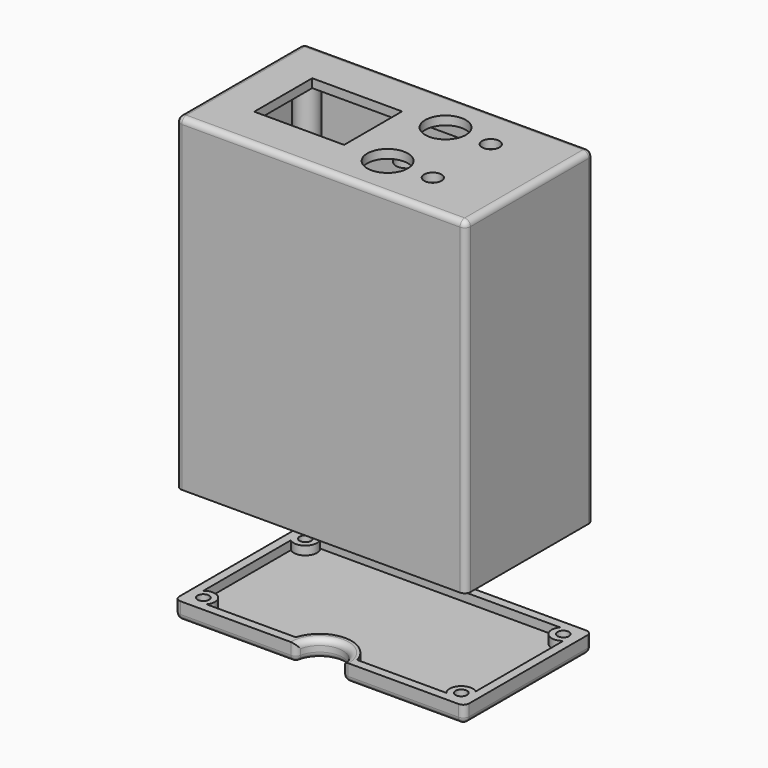
from build123d import *

# Parameters (mm, degrees)
F0_W      = 100
F0_H      = 55
F0_R      = 2.5
F0_R_2    = 7
F0_R_3    = 3
F0_W_2    = 31
F0_H_2    = 25
F1_DEPTH  = 3
F2_DEPTH  = 110
F3_R      = 3.5
F3_R_2    = 1.5
F3_W      = 49.6577308513
F3_H      = 4
F3_R_3    = 1
F4_DEPTH  = 4
F5_R      = 2
F7_R      = 3
F8_DEPTH  = 3
F7_R_2    = 2
F9_DEPTH  = 6
F11_DEPTH = 2.9
F12_R     = 2


# Not quite as in the source:
# - a feature of the source that left no trace in its solid (it failed there, or was rolled back) is left out
# - a feature names something its author has since deleted; it is built from what else it names


with BuildPart() as f1:
    # F0 (on Top) → F1 (new body)
    with BuildSketch(Plane.XY):
        Rectangle(F0_W, F0_H)
        with Locations((-44.5, -22)):
            Circle(F0_R, mode=Mode.SUBTRACT)
        with Locations((44.5, -22)):
            Circle(F0_R, mode=Mode.SUBTRACT)
        with Locations((-44.5, 22)):
            Circle(F0_R, mode=Mode.SUBTRACT)
        with BuildLine():
            ThreePointArc((-47, 18.8775010008), (-41.6715728753, 19.1715728753), (-41.3775010008, 24.5))
            Line((-41.3775010008, 24.5), (41.3775010008, 24.5))
            ThreePointArc((41.3775010008, 24.5), (41.6715728753, 19.1715728753), (47, 18.8775010008))
            Line((47, 18.8775010008), (47, -18.8775010008))
            ThreePointArc((47, -18.8775010008), (41.6715728753, -19.1715728753), (41.3775010008, -24.5))
            Line((41.3775010008, -24.5), (-41.3775010008, -24.5))
            ThreePointArc((-41.3775010008, -24.5), (-41.6715728753, -19.1715728753), (-47, -18.8775010008))
            Line((-47, -18.8775010008), (-47, 18.8775010008))
        make_face(mode=Mode.SUBTRACT)
        with Locations((44.5, 22)):
            Circle(F0_R, mode=Mode.SUBTRACT)
        with BuildLine():
            Line((41.3775010008, 24.5), (-41.3775010008, 24.5))
            ThreePointArc((-41.3775010008, 24.5), (-41.6715728753, 19.1715728753), (-47, 18.8775010008))
            Line((-47, 18.8775010008), (-47, -18.8775010008))
            ThreePointArc((-47, -18.8775010008), (-41.6715728753, -19.1715728753), (-41.3775010008, -24.5))
            Line((-41.3775010008, -24.5), (41.3775010008, -24.5))
            ThreePointArc((41.3775010008, -24.5), (41.6715728753, -19.1715728753), (47, -18.8775010008))
            Line((47, -18.8775010008), (47, 18.8775010008))
            ThreePointArc((47, 18.8775010008), (41.6715728753, 19.1715728753), (41.3775010008, 24.5))
        make_face()
        with Locations((11, -12.5)):
            Circle(F0_R_2, mode=Mode.SUBTRACT)
        with Locations((26.6150971745, -12.5)):
            Circle(F0_R_3, mode=Mode.SUBTRACT)
        with Locations((-19.5, 0)):
            Rectangle(F0_W_2, F0_H_2, mode=Mode.SUBTRACT)
        with Locations((11, 12.5)):
            Circle(F0_R_2, mode=Mode.SUBTRACT)
        with Locations((26.6150971745, 12.5)):
            Circle(F0_R_3, mode=Mode.SUBTRACT)
        with Locations((-44.5, 22)):
            Circle(F0_R)
        with Locations((-44.5, -22)):
            Circle(F0_R)
        with Locations((44.5, -22)):
            Circle(F0_R)
        with Locations((44.5, 22)):
            Circle(F0_R)
    extrude(amount=F1_DEPTH)

    # F0 (on Top) → F2 (join)
    with BuildSketch(Plane.XY):
        Rectangle(F0_W, F0_H)
        with Locations((-44.5, -22)):
            Circle(F0_R, mode=Mode.SUBTRACT)
        with Locations((44.5, -22)):
            Circle(F0_R, mode=Mode.SUBTRACT)
        with Locations((-44.5, 22)):
            Circle(F0_R, mode=Mode.SUBTRACT)
        with BuildLine():
            ThreePointArc((-47, 18.8775010008), (-41.6715728753, 19.1715728753), (-41.3775010008, 24.5))
            Line((-41.3775010008, 24.5), (41.3775010008, 24.5))
            ThreePointArc((41.3775010008, 24.5), (41.6715728753, 19.1715728753), (47, 18.8775010008))
            Line((47, 18.8775010008), (47, -18.8775010008))
            ThreePointArc((47, -18.8775010008), (41.6715728753, -19.1715728753), (41.3775010008, -24.5))
            Line((41.3775010008, -24.5), (-41.3775010008, -24.5))
            ThreePointArc((-41.3775010008, -24.5), (-41.6715728753, -19.1715728753), (-47, -18.8775010008))
            Line((-47, -18.8775010008), (-47, 18.8775010008))
        make_face(mode=Mode.SUBTRACT)
        with Locations((44.5, 22)):
            Circle(F0_R, mode=Mode.SUBTRACT)
    extrude(amount=-F2_DEPTH)

    # F3 (on face) → F4 (join)
    with BuildSketch(Plane.XY):
        with Locations((37, 0.5)):
            Circle(F3_R)
        with Locations((37, 0.5)):
            Circle(F3_R_2, mode=Mode.SUBTRACT)
        with Locations((7, 0.5)):
            Circle(F3_R)
        with Locations((7, 0.5)):
            Circle(F3_R_2, mode=Mode.SUBTRACT)
        with Locations((-10.6749895494, 22.5)):
            Rectangle(F3_W, F3_H)
        with Locations((-2.5, 22.5)):
            Circle(F3_R_3, mode=Mode.SUBTRACT)
    extrude(amount=-F4_DEPTH)

    # F5
    f5_edges = [f1.edges().sort_by_distance(p)[0] for p in [
        (50, 27.5, -53.5),
        (-50, 27.5, -53.5),
        (-50, -27.5, -53.5),
        (50, -27.5, -53.5),
        (0, 27.5, 3),
        (-50, 0, 3),
        (0, -27.5, 3),
        (50, 0, 3),
    ]]
    fillet(f5_edges, radius=F5_R)


with BuildPart() as f8:
    # F7 (on offset) → F8 (new body)
    with BuildSketch(Plane.XY.offset(-150)):
        with BuildLine():
            Line((49.5320752355, 27.5), (-50.4679247645, 27.5))
            Line((-50.4679247645, 27.5), (-50.4679247645, -27.5))
            Line((-50.4679247645, -27.5), (-8.4679247645, -27.5))
            ThreePointArc((-8.4679247645, -27.5), (-0.4679247645, -19.5), (7.5320752355, -27.5))
            Line((7.5320752355, -27.5), (49.5320752355, -27.5))
            Line((49.5320752355, -27.5), (49.5320752355, 27.5))
        make_face()
        with Locations((-44.9679247645, -22)):
            Circle(F7_R, mode=Mode.SUBTRACT)
        with Locations((44.0320752355, -22)):
            Circle(F7_R, mode=Mode.SUBTRACT)
        with Locations((-44.9679247645, 22)):
            Circle(F7_R, mode=Mode.SUBTRACT)
        with BuildLine():
            ThreePointArc((-47.4679247645, 18.8775010008), (-42.1394976398, 19.1715728753), (-41.8454257653, 24.5))
            Line((-41.8454257653, 24.5), (40.9095762363, 24.5))
            ThreePointArc((40.9095762363, 24.5), (41.2036481107, 19.1715728753), (46.5320752355, 18.8775010008))
            Line((46.5320752355, 18.8775010008), (46.5320752355, -18.8775010008))
            ThreePointArc((46.5320752355, -18.8775010008), (41.2036481107, -19.1715728753), (40.9095762363, -24.5))
            Line((40.9095762363, -24.5), (10.1150804797, -24.5))
            ThreePointArc((10.1150804797, -24.5), (-0.4679247645, -16.5), (-11.0509300088, -24.5))
            Line((-11.0509300088, -24.5), (-41.8454257653, -24.5))
            ThreePointArc((-41.8454257653, -24.5), (-42.1394976398, -19.1715728753), (-47.4679247645, -18.8775010008))
            Line((-47.4679247645, -18.8775010008), (-47.4679247645, 18.8775010008))
        make_face(mode=Mode.SUBTRACT)
        with Locations((44.0320752355, 22)):
            Circle(F7_R, mode=Mode.SUBTRACT)
        with BuildLine():
            Line((40.9095762363, 24.5), (-41.8454257653, 24.5))
            ThreePointArc((-41.8454257653, 24.5), (-42.1394976398, 19.1715728753), (-47.4679247645, 18.8775010008))
            Line((-47.4679247645, 18.8775010008), (-47.4679247645, -18.8775010008))
            ThreePointArc((-47.4679247645, -18.8775010008), (-42.1394976398, -19.1715728753), (-41.8454257653, -24.5))
            Line((-41.8454257653, -24.5), (-11.0509300088, -24.5))
            ThreePointArc((-11.0509300088, -24.5), (-0.4679247645, -16.5), (10.1150804797, -24.5))
            Line((10.1150804797, -24.5), (40.9095762363, -24.5))
            ThreePointArc((40.9095762363, -24.5), (41.2036481107, -19.1715728753), (46.5320752355, -18.8775010008))
            Line((46.5320752355, -18.8775010008), (46.5320752355, 18.8775010008))
            ThreePointArc((46.5320752355, 18.8775010008), (41.2036481107, 19.1715728753), (40.9095762363, 24.5))
        make_face()
    extrude(amount=F8_DEPTH)

    # F7 (on offset) → F9 (join)
    with BuildSketch(Plane.XY.offset(-150)):
        with BuildLine():
            Line((49.5320752355, 27.5), (-50.4679247645, 27.5))
            Line((-50.4679247645, 27.5), (-50.4679247645, -27.5))
            Line((-50.4679247645, -27.5), (-8.4679247645, -27.5))
            ThreePointArc((-8.4679247645, -27.5), (-0.4679247645, -19.5), (7.5320752355, -27.5))
            Line((7.5320752355, -27.5), (49.5320752355, -27.5))
            Line((49.5320752355, -27.5), (49.5320752355, 27.5))
        make_face()
        with Locations((-44.9679247645, -22)):
            Circle(F7_R, mode=Mode.SUBTRACT)
        with Locations((44.0320752355, -22)):
            Circle(F7_R, mode=Mode.SUBTRACT)
        with Locations((-44.9679247645, 22)):
            Circle(F7_R, mode=Mode.SUBTRACT)
        with BuildLine():
            ThreePointArc((-47.4679247645, 18.8775010008), (-42.1394976398, 19.1715728753), (-41.8454257653, 24.5))
            Line((-41.8454257653, 24.5), (40.9095762363, 24.5))
            ThreePointArc((40.9095762363, 24.5), (41.2036481107, 19.1715728753), (46.5320752355, 18.8775010008))
            Line((46.5320752355, 18.8775010008), (46.5320752355, -18.8775010008))
            ThreePointArc((46.5320752355, -18.8775010008), (41.2036481107, -19.1715728753), (40.9095762363, -24.5))
            Line((40.9095762363, -24.5), (10.1150804797, -24.5))
            ThreePointArc((10.1150804797, -24.5), (-0.4679247645, -16.5), (-11.0509300088, -24.5))
            Line((-11.0509300088, -24.5), (-41.8454257653, -24.5))
            ThreePointArc((-41.8454257653, -24.5), (-42.1394976398, -19.1715728753), (-47.4679247645, -18.8775010008))
            Line((-47.4679247645, -18.8775010008), (-47.4679247645, 18.8775010008))
        make_face(mode=Mode.SUBTRACT)
        with Locations((44.0320752355, 22)):
            Circle(F7_R, mode=Mode.SUBTRACT)
        with Locations((-44.9679247645, -22)):
            Circle(F7_R)
        with Locations((-44.9679247645, -22)):
            Circle(F7_R_2, mode=Mode.SUBTRACT)
        with Locations((-44.9679247645, 22)):
            Circle(F7_R)
        with Locations((-44.9679247645, 22)):
            Circle(F7_R_2, mode=Mode.SUBTRACT)
        with Locations((44.0320752355, 22)):
            Circle(F7_R)
        with Locations((44.0320752355, 22)):
            Circle(F7_R_2, mode=Mode.SUBTRACT)
        with Locations((44.0320752355, -22)):
            Circle(F7_R)
        with Locations((44.0320752355, -22)):
            Circle(F7_R_2, mode=Mode.SUBTRACT)
    extrude(amount=F9_DEPTH)

    # F7 (on offset) → F11 (cut)
    with BuildSketch(Plane.XY.offset(-150)):
        with Locations((-44.9679247645, 22)):
            Circle(F7_R)
        with Locations((-44.9679247645, 22)):
            Circle(F7_R_2, mode=Mode.SUBTRACT)
        with Locations((44.0320752355, 22)):
            Circle(F7_R)
        with Locations((44.0320752355, 22)):
            Circle(F7_R_2, mode=Mode.SUBTRACT)
        with Locations((44.0320752355, -22)):
            Circle(F7_R)
        with Locations((44.0320752355, -22)):
            Circle(F7_R_2, mode=Mode.SUBTRACT)
        with Locations((-44.9679247645, -22)):
            Circle(F7_R)
        with Locations((-44.9679247645, -22)):
            Circle(F7_R_2, mode=Mode.SUBTRACT)
    extrude(amount=F11_DEPTH, mode=Mode.SUBTRACT)

    # F12
    f12_edges = [f8.edges().sort_by_distance(p)[0] for p in [
        (-50.467925, -27.5, -147),
        (-50.467925, 27.5, -147),
        (49.532075, 27.5, -147),
        (49.532075, 0, -150),
        (-29.467925, -27.5, -150),
        (-50.467925, 0, -150),
        (-0.467925, 27.5, -150),
        (7.532075, -27.5, -147),
        (28.532075, -27.5, -150),
        (-0.467925, -19.5, -150),
        (-0.467925, -19.5, -144),
        (49.532075, -27.5, -147),
        (-8.467925, -27.5, -147),
    ]]
    fillet(f12_edges, radius=F12_R)


solid = Compound([f1.part, f8.part])
